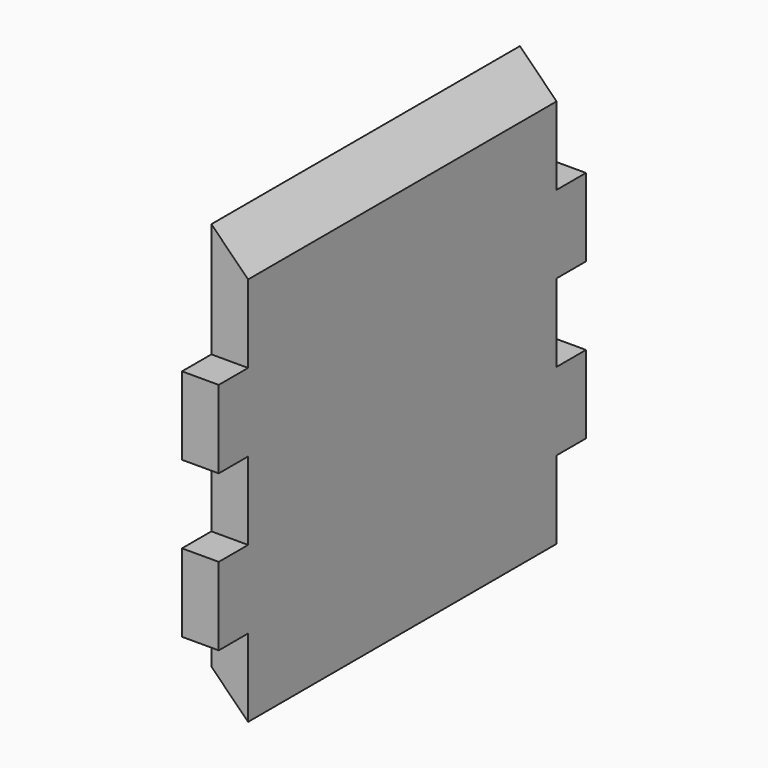
from build123d import *

# Parameters (mm, degrees)
F2_W     = 250
F2_H     = 232.13203
F3_DEPTH = 10
F5_DEPTH = 125
F6_W     = 20
F6_H     = 42.426406
F7_DEPTH = 20


# Not quite as in the source:
# - a pattern or mirror of a feature is missing from the dataset's text; its kind, count and spacing are read off the source's solid


with BuildPart() as f3:
    # F2 (on Right) → F3 (new body, symmetric)
    with BuildSketch(Plane.YZ):
        Rectangle(F2_W, F2_H)
    extrude(amount=F3_DEPTH, both=True)

    # F4 (on Front) → F5 (cut, symmetric)
    with BuildSketch(Plane.XZ):
        Polygon((10, 116.066015), (-10, 116.066015), (10, 96.066015), align=None)
        Polygon((-10, -116.066015), (10, -116.066015), (-10, -96.066015), align=None)
    extrude(amount=F5_DEPTH, both=True, mode=Mode.SUBTRACT)

    # F6 (on face) → F7 (cut)
    with BuildSketch(Plane.XZ.offset(125)):
        Polygon((-10, 53.639609), (10, 53.639609), (10, 96.066015), (-10, 116.066015), (-10, 96.066015), align=None)
        with Locations((0, -10)):
            Rectangle(F6_W, F6_H)
        with Locations((0, -94.852812)):
            Rectangle(F6_W, F6_H)
    f7 = extrude(amount=-F7_DEPTH, mode=Mode.SUBTRACT)

    # F7_copies: F7 across plane
    add(f7.mirror(Plane.ZX), mode=Mode.SUBTRACT)


solid = f3.part
